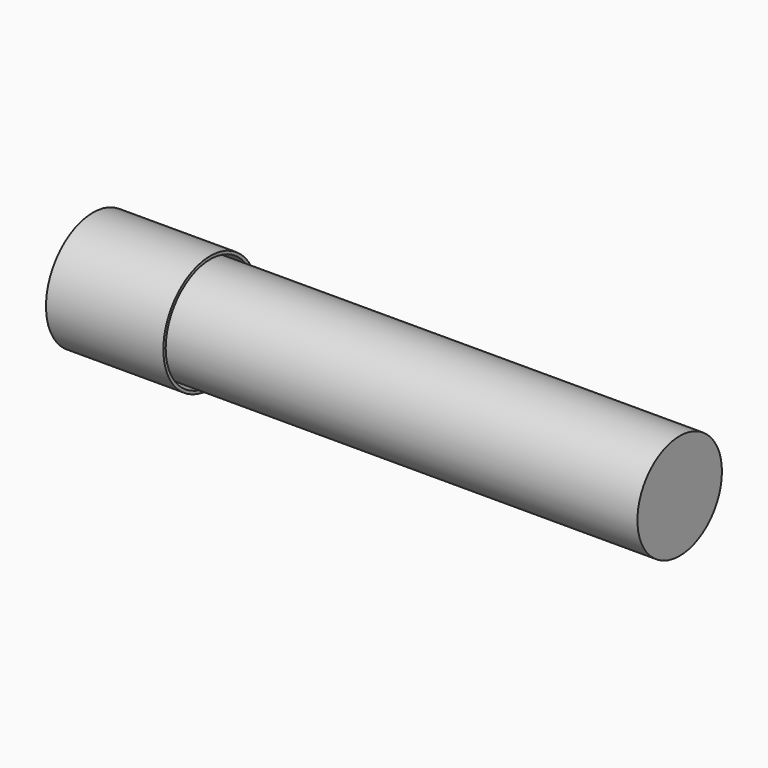
from build123d import *

# Parameters (mm, degrees)
F0_R     = 12.7
F1_DEPTH = 25.4
F3_D     = 24.13
F4_R     = 11.43
F5_DEPTH = 127


# Not quite as in the source:
# - the program builds the solid bodies; features that only make, move or delete a surface that nothing else refers to are left out


with BuildPart() as f1:
    # F0 (on Right) → F1 (new body)
    with BuildSketch(Plane.YZ):
        Circle(F0_R)
    extrude(amount=F1_DEPTH)

    # F3 (through all)
    with Locations(Plane.YZ.offset(25.4)):
        with Locations((0, 0)):
            Hole(F3_D / 2)


with BuildPart() as f5:
    # F4 (on Right) → F5 (new body)
    with BuildSketch(Plane.YZ):
        Circle(F4_R)
    extrude(amount=F5_DEPTH)


solid = Compound([f1.part, f5.part])
